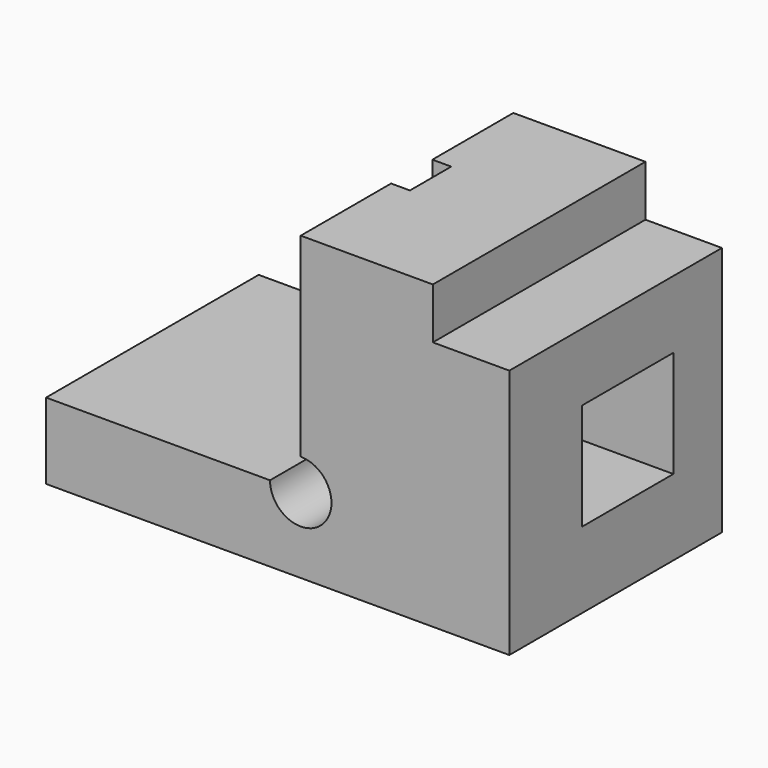
from build123d import *

# Parameters (mm, degrees)
F0_W           = 61.9914149866
F0_H           = 40.331762284
F1_DEPTH       = 20.32
F2_DEPTH       = 15.24
F5_R           = 4.1121060328
F6_DEPTH       = 20.32
F7_W           = 14.0040833503
F7_H           = 6.9086803123
F8_DEPTH       = 17.78
F9_W           = 15.3111321852
F9_H           = 14.2841655761
F10_DEPTH      = 61.9924149866
F10_DEPTH_BACK = 25.4
F11_W          = 10.2332767595
F11_H          = 6.8242249937
F12_DEPTH      = 35.561
F13_W          = 34.0766059235
F13_H          = 30.1554612815
F14_DEPTH      = 35.561


# Not quite as in the source:
# - the program builds the solid bodies; features that only make, move or delete a surface that nothing else refers to are left out


with BuildPart() as f1:
    # F0 (on Front) → F1 (new body)
    with BuildSketch(Plane.XZ):
        with Locations((-3.0808984302, 9.9895801395)):
            Rectangle(F0_W, F0_H)
    extrude(amount=F1_DEPTH)

    # F2 (add): a face of the model
    f2_faces = [f1.faces().sort_by_distance(p)[0] for p in [
        (-3.0808984302, -20.32, 9.9895801395),
    ]]
    extrude(f2_faces, amount=F2_DEPTH)

    # F5 (on face) → F6 (cut)
    with BuildSketch(Plane.XZ.offset(35.56)):
        Circle(F5_R)
    extrude(amount=-F6_DEPTH, mode=Mode.SUBTRACT)

    # F7 (on face) → F8 (cut)
    with BuildSketch(Plane.XY.offset(30.1554612815)):
        with Locations((-4.4813072309, -16.991621349)):
            Rectangle(F7_W, F7_H)
    extrude(amount=-F8_DEPTH, mode=Mode.SUBTRACT)

    # F9 (on face) → F10 (cut, two sides)
    with BuildSketch(Plane.YZ.offset(27.9148090631)) as f10_sk:
        with Locations((-15.7779348083, 7.1420827881)):
            Rectangle(F9_W, F9_H)
    extrude(amount=-F10_DEPTH, mode=Mode.SUBTRACT)
    extrude(f10_sk.sketch, amount=F10_DEPTH_BACK, mode=Mode.SUBTRACT)

    # F11 (on face) → F12 (cut, through all)
    with BuildSketch(Plane.XZ.offset(35.56)):
        with Locations((22.7981706833, 26.7433487847)):
            Rectangle(F11_W, F11_H)
    extrude(amount=-F12_DEPTH, mode=Mode.SUBTRACT)

    # F13 (on face) → F14 (cut, through all)
    with BuildSketch(Plane.XZ):
        with Locations((-17.0383029617, 15.0777306408)):
            Rectangle(F13_W, F13_H)
    extrude(amount=F14_DEPTH, mode=Mode.SUBTRACT)


solid = f1.part
